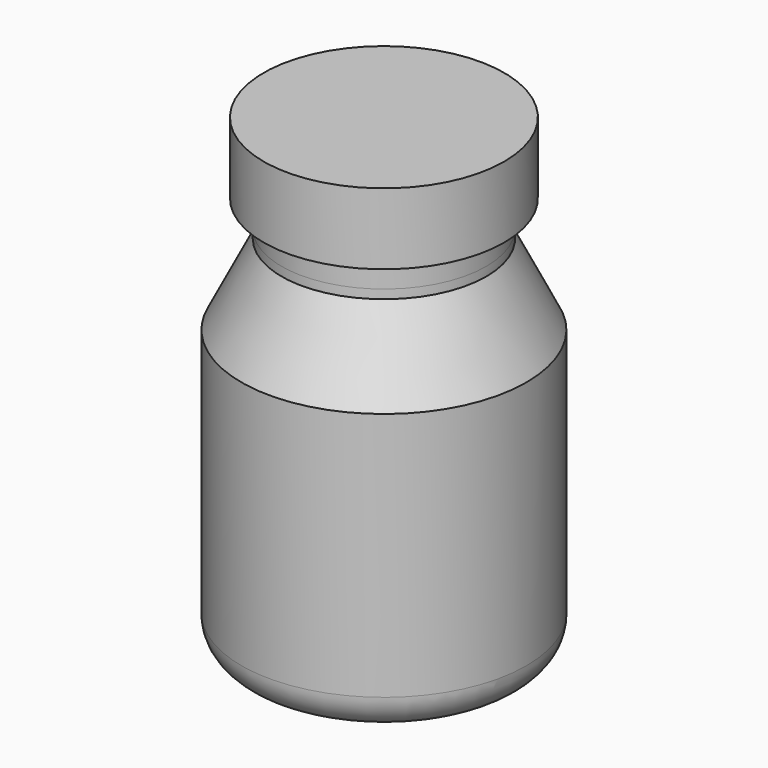
from build123d import *

# Parameters (mm, degrees)
F0_R        = 25.4
F0_R_2      = 21.43125
F0_R_3      = 18.25625
F1_DEPTH    = 66.675
F2_DEPTH    = 84.1375
F3_R        = 6.35
F4_S5_R     = 18.25625
F4_T6_DEPTH = 38
F5_START    = 71.4375
F5_DEPTH    = 12.7


# Not quite as in the source:
# - a fillet or chamfer that OpenCascade refuses, or shapes differently, is made with other operations: its cross-section is extruded or revolved along the edge and cut away or added


with BuildPart() as f1:
    # F0 (on Top) → F1 (new body)
    with BuildSketch(Plane.XY):
        Circle(F0_R)
        Circle(F0_R_2, mode=Mode.SUBTRACT)
        Circle(F0_R_2)
        Circle(F0_R_3, mode=Mode.SUBTRACT)
    extrude(amount=F1_DEPTH)

    # F0 (on Top) → F2 (join)
    with BuildSketch(Plane.XY):
        Circle(F0_R_3)
    extrude(amount=F2_DEPTH)

    # F3
    f3_edges = [f1.edges().sort_by_distance(p)[0] for p in [
        (-25.4, 0, 0),
    ]]
    fillet(f3_edges, radius=F3_R)

    # F4: chamfer of 7.9375 x 15.875 on 1 edges, made by hand


with BuildPart() as f4_tool2:
    # F4_s3 → F4_t4 (revolve)
    with BuildSketch(Plane.XZ):
        Polygon((25.4, 50.8), (17.4625, 66.675), (25.4, 66.675), align=None)
    revolve(axis=Axis((0, 0, 66.675), (0, 0, 1)))

    # F4_s5 → F4_t6 (cut, symmetric)
    with BuildSketch(Plane.XY.offset(58.7)):
        Circle(F4_S5_R)
    extrude(amount=F4_T6_DEPTH, both=True, mode=Mode.SUBTRACT)


with BuildPart() as f1_1:
    add(f1.part)

    # F4_t1: cut F4_tool2
    add(f4_tool2.part, mode=Mode.SUBTRACT)

    # F0 (on Top) → F5 (join)
    with BuildSketch(Plane.XY.offset(F5_START)):
        Circle(F0_R_2)
        Circle(F0_R_3, mode=Mode.SUBTRACT)
    extrude(amount=F5_DEPTH)


solid = f1_1.part
